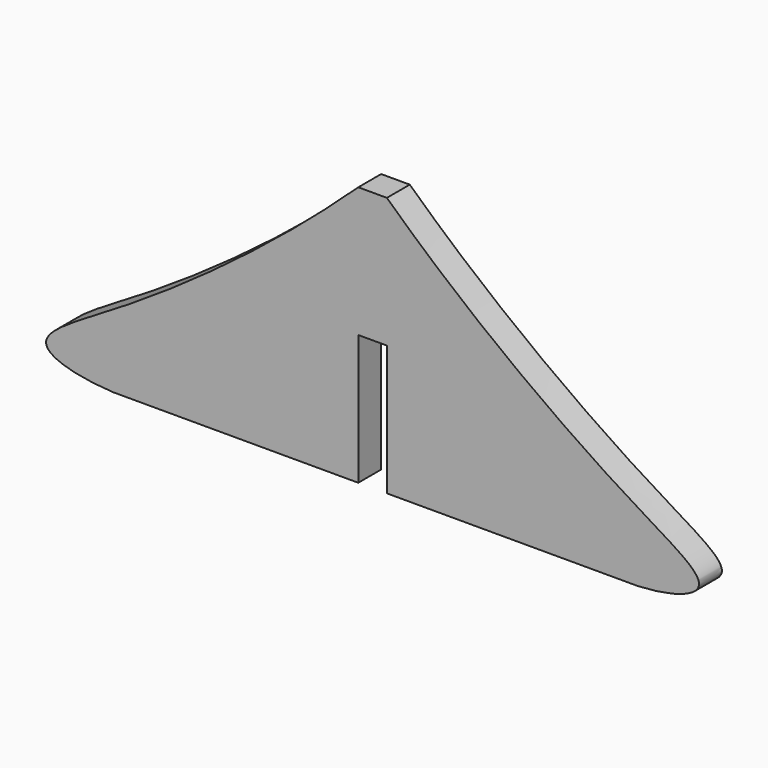
from build123d import *

# Parameters (mm, degrees)
F1_DEPTH = 5.588


with BuildPart() as f1:
    # F0 (on Front) → F1 (new body)
    with BuildSketch(Plane.XZ):
        with BuildLine():
            add(Edge.make_bspline(
                [(59.2453815043, 135.979577899), (52.4327556863, 136.2949171435), (39.9709976325, 139.4898068104), (63.9913458796, 152.1116502589), (90.2434246222, 171.0211149335), (107.0472194433, 186.7697834969)],
                knots=[0, 0, 0, 0, 0.2385633235, 0.5008288966, 1, 1, 1, 1], degree=3))
            Line((59.2453815043, 135.979577899), (107.0472194433, 135.979577899))
            Line((107.0472194433, 135.979577899), (107.0472194433, 161.379577899))
            Line((107.0472194433, 161.379577899), (112.6352194433, 161.379577899))
            Line((112.6352194433, 161.379577899), (112.6352194433, 135.979577899))
            Line((112.6352194433, 135.979577899), (161.6750980084, 135.979577899))
            add(Edge.make_bspline(
                [(161.6750980084, 135.979577899), (168.2971610007, 136.2860964716), (178.8323776641, 139.7062489389), (157.2734114026, 151.2672606436), (129.9250364204, 170.5656105709), (112.6352194433, 186.7697834969)],
                knots=[0, 0, 0, 0, 0.2318902282, 0.4863911926, 1, 1, 1, 1], degree=3))
            Line((112.6352194433, 186.7697834969), (107.0472194433, 186.7697834969))
        make_face()
    extrude(amount=F1_DEPTH)


solid = f1.part
